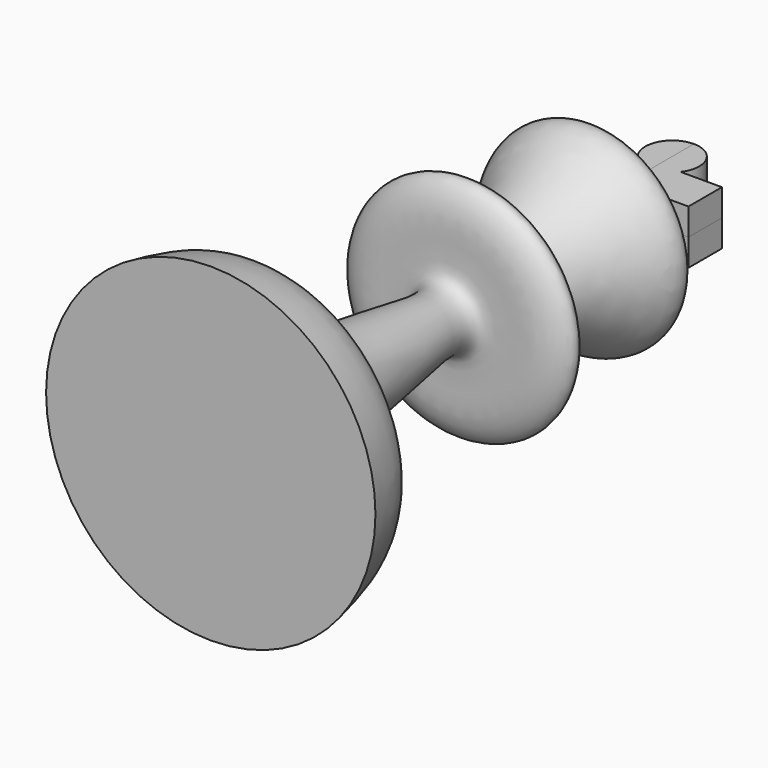
from build123d import *

# Parameters (mm, degrees)
F3_DEPTH = 2.54


with BuildPart() as f1:
    # F0 (on Top) → F1 (revolve)
    with BuildSketch(Plane.XY):
        with BuildLine():
            Line((0, 44.9221981495), (0, 0))
            Line((0, 0), (15.494, 0))
            add(Edge.make_bspline(
                [(0, 44.9221981495), (3.736772829, 45.336830534), (9.2662334796, 45.9620664317), (9.5318619851, 43.0548774337), (7.4647608952, 40.3291635776), (6.0871811267, 37.6427233499), (4.8332844055, 34.6072404278), (4.0802391458, 30.4466318813), (8.4114159869, 31.7824023444), (11.8039739097, 29.7365303211), (8.1592319875, 27.3457479457), (1.7130923926, 28.9811819361), (3.5861831087, 21.3705978805), (4.5811585373, 8.9378626053), (9.6930172716, 6.6582013987), (14.4132171946, 6.2120398673), (15.0969928272, 1.9154757576), (15.494, 0)],
                knots=[0, 0, 0, 0, 0.0943864096, 0.1359623409, 0.1941000917, 0.2497326581, 0.3095822178, 0.3637547274, 0.4235014961, 0.475780506, 0.5307638211, 0.6018151135, 0.6784266289, 0.7909617911, 0.8604296571, 0.9240567804, 1, 1, 1, 1], degree=3))
        make_face()
    revolve(axis=Axis((0, 22.4610990748, 0), (0, 1, 0)))


with BuildPart() as f3:
    # F2 (on Top) → F3 (new body)
    with BuildSketch(Plane.XY):
        with BuildLine():
            Line((-2.0178398117, 48.7928502262), (-3.81, 45.4306691097))
            Line((-3.81, 45.4306691097), (0, 45.4306691097))
            Line((0, 45.4306691097), (0, 56.8125499682))
            ThreePointArc((0, 56.8125499682), (-2.2770658033, 55.3979704797), (-2.0178398117, 52.7298502262))
            Line((-2.0178398117, 52.7298502262), (-5.9055439197, 52.7298502262))
            Line((-5.9055439197, 52.7298502262), (-5.9055439197, 48.7928502262))
            Line((-5.9055439197, 48.7928502262), (-2.0178398117, 48.7928502262))
        make_face()
    extrude(amount=F3_DEPTH)


with BuildPart() as f4_1:
    # F4: instance of F3
    add(f3.part.mirror(Plane.YZ))


with BuildPart() as f5_1:
    # F5: instance of F4_1
    add(f4_1.part.mirror(Plane.XY))


with BuildPart() as f5_2:
    # F5: instance of F3
    add(f3.part.mirror(Plane.XY))


solid = Compound([f1.part, f3.part, f4_1.part, f5_1.part, f5_2.part])
